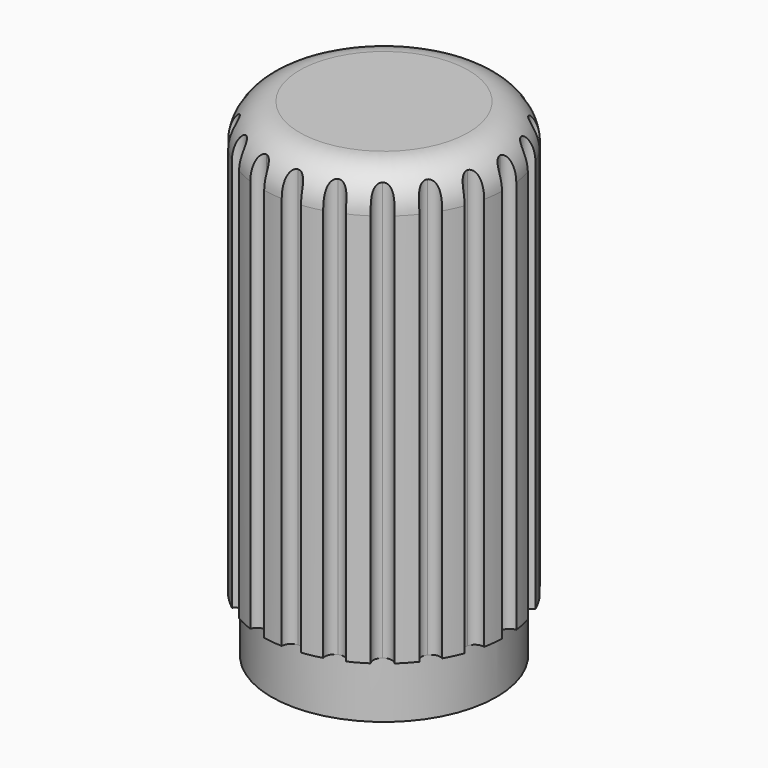
from build123d import *

# Parameters (mm, degrees)
F2_R            = 2
F4_DEPTH        = 22.3238757488
F4_COPIES_COUNT = 20


# Not quite as in the source:
# - a pattern or mirror of a feature is missing from the dataset's text; its kind, count and spacing are read off the source's solid


with BuildPart() as f1:
    # F0 (on Front) → F1 (revolve)
    with BuildSketch(Plane.XZ):
        Polygon((-27.0206088985, 40.1582903922), (-27.0206088985, 37.1582903922), (-22.9206088985, 37.1582903922), (-22.9206088985, 14.1582903922), (-21.0206088985, 14.1582903922), (-21.0206088985, 17.1582903922), (-20.5206088985, 17.1582903922), (-20.5206088985, 40.1582903922), align=None)
    revolve(axis=Axis((-27.0206088985, 0, 38.6582903922), (0, 0, 1)))

    # F2
    f2_edges = [f1.edges().sort_by_distance(p)[0] for p in [
        (-33.520609, 0, 40.15829),
    ]]
    fillet(f2_edges, radius=F2_R)

    # F3 (on face) → F4 (cut, through all)
    with BuildSketch(Plane(origin=(0, 0, 17.1582903922), x_dir=(1, 0, 0), z_dir=(0, 0, -1))):
        with BuildLine():
            ThreePointArc((-24.3191343217, 5.9120246203), (-24.781561481, 6.1021854005), (-25.2572374416, 6.2562385748))
            ThreePointArc((-25.2572374416, 6.2562385748), (-25.2311391408, 5.8833705751), (-24.9537958637, 5.6327865111))
            ThreePointArc((-24.9537958637, 5.6327865111), (-24.5802000092, 5.6445244369), (-24.3191343217, 5.9120246203))
        make_face()
    f4 = extrude(amount=-F4_DEPTH, mode=Mode.SUBTRACT)

    # F4_copies: F4 ×20 about axis
    f4_copies_axis = Axis((-27.020609, 1e-06, 0), (0, 0, 1))
    for i in range(1, F4_COPIES_COUNT):
        add(f4.rotate(f4_copies_axis, i * 360 / F4_COPIES_COUNT), mode=Mode.SUBTRACT)


solid = f1.part
